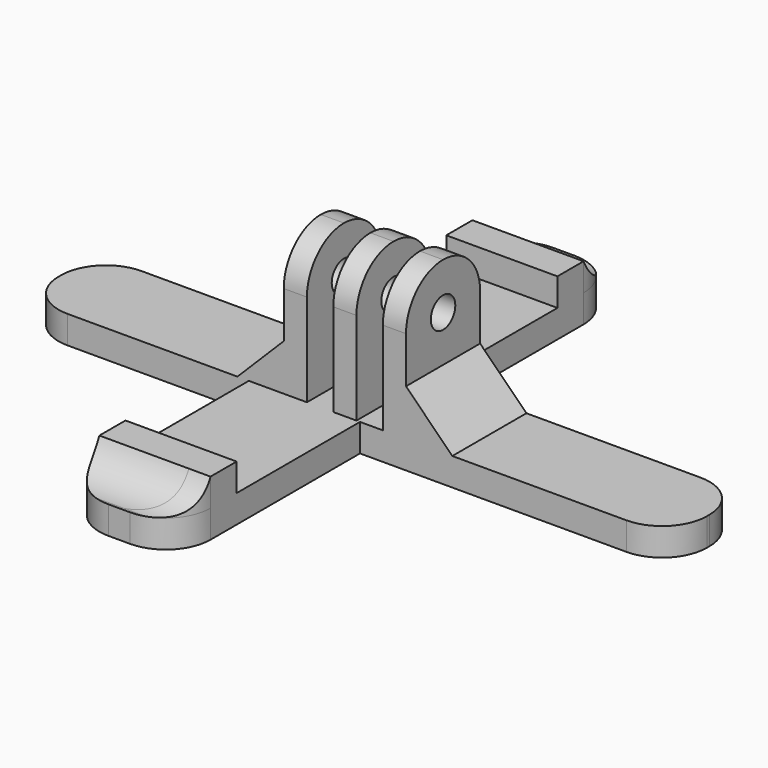
from build123d import *

# Parameters (mm, degrees)
F0_W          = 12
F0_H          = 25
F1_DEPTH      = 3
F2_W          = 2.5
F2_H          = 10
F3_DEPTH      = 15
F5_D          = 3.3
F6_R          = 4.99999
F7_R          = 4.8284271247
F8_T1_DEPTH   = 10
F9_W          = 12
F9_H          = 3.5225884728
F10_DEPTH     = 3
F11_T3_DEPTH  = 34.9128784748
F11_S4_R      = 4.8284271247
F11_T5_DEPTH  = 19
F11_T8_DEPTH  = 34.9128784748
F11_S9_R      = 4.8284271247
F11_T10_DEPTH = 19
F11_T13_DEPTH = 34.9128784748
F11_S14_R     = 4.8284271247
F11_T15_DEPTH = 19
F11_T18_DEPTH = 34.9128784748
F11_S19_R     = 4.8284271247
F11_T20_DEPTH = 19


# Not quite as in the source:
# - a fillet or chamfer that OpenCascade refuses, or shapes differently, is made with other operations: its cross-section is extruded or revolved along the edge and cut away or added
# - a fillet or chamfer is up to 0.001 mm smaller than in the source, because OpenCascade refuses the exact size


with BuildPart() as f1:
    # F0 (on Top) → F1 (new body)
    with BuildSketch(Plane.XY):
        Polygon((35, -5), (35, 5), (1.4061683491, 5), (-10.5938316509, 5), (-35, 5), (-35, -5), (-10.5938316509, -5), (1.4061683491, -5), align=None)
        with Locations((-4.5938316509, 17.5)):
            Rectangle(F0_W, F0_H)
        with Locations((-4.5938316509, -17.5)):
            Rectangle(F0_W, F0_H)
    extrude(amount=F1_DEPTH)

    # F2 (on face) → F3 (join)
    with BuildSketch(Plane.XY.offset(3)):
        with Locations((-5.5737404495, 0)):
            Rectangle(F2_W, F2_H)
        with Locations((-0.2237404495, 0)):
            Rectangle(F2_W, F2_H)
        with Locations((5.1262595505, 0)):
            Rectangle(F2_W, F2_H)
    extrude(amount=F3_DEPTH)

    # F5 (through all)
    with Locations(Plane.YZ.offset(6.3762595505)):
        with Locations((0, 12.9813589156)):
            Hole(F5_D / 2)

    # F6 (radius 5 in the source; OpenCascade refuses exactly that, so slightly less here)
    f6_edges = [f1.edges().sort_by_distance(p)[0] for p in [
        (5.12626, 5, 18),
        (-0.22374, 5, 18),
        (-5.57374, 5, 18),
        (-5.57374, -5, 18),
        (-0.22374, -5, 18),
        (5.12626, -5, 18),
    ]]
    fillet(f6_edges, radius=F6_R)

    # F7
    f7_edges = [f1.edges().sort_by_distance(p)[0] for p in [
        (35, 5, 1.5),
        (35, -5, 1.5),
        (-35, -5, 1.5),
        (-35, 5, 1.5),
        (-10.593832, -30, 1.5),
        (1.406168, -30, 1.5),
        (1.406168, 30, 1.5),
        (-10.593832, 30, 1.5),
    ]]
    fillet(f7_edges, radius=F7_R)

    # F8: chamfer of 5 on 2 edges, made by hand

    # F8_s2 → F8_t1 (join)
    with BuildSketch(Plane.XZ.offset(-5)):
        Polygon((11.3762595505, 3), (6.3762595505, 8), (6.3762595505, 3), align=None)
        Polygon((-11.8237404495, 3), (-6.8237404495, 8), (-6.8237404495, 3), align=None)
    extrude(amount=F8_T1_DEPTH)

    # F9 (on face) → F10 (join)
    with BuildSketch(Plane.XY.offset(3)):
        with Locations((-4.5938316509, 23.4102786388)):
            Rectangle(F9_W, F9_H)
        with Locations((-4.5938316509, -23.4102786388)):
            Rectangle(F9_W, F9_H)
    extrude(amount=F10_DEPTH)

    # F11: fillet of radius 5 on 2 edges, made by hand


with BuildPart() as f11_tool1:
    # F11_s2 → F11_t3 (new body)
    with BuildSketch(Plane.YZ.offset(-22.0502708883)):
        with BuildLine():
            ThreePointArc((-29.7541485702, 3), (-27.0155357827, 3.8166998673), (-25.1715728753, 6))
            Line((-25.1715728753, 6), (-25.1715728753, 3))
            Line((-25.1715728753, 3), (-29.7541485702, 3))
        make_face()
    extrude(amount=F11_T3_DEPTH)

    # F11_s4 → F11_t5 (intersect, symmetric)
    with BuildSketch(Plane.XY.offset(4.5)):
        with Locations((-5.7654045262, -25.1715728753)):
            Circle(F11_S4_R)
    extrude(amount=F11_T5_DEPTH, both=True, mode=Mode.INTERSECT)


with BuildPart() as f11_tool6:
    # F11_s7 → F11_t8 (new body)
    with BuildSketch(Plane.YZ.offset(-22.0502708883)):
        with BuildLine():
            ThreePointArc((-29.7541485702, 3), (-27.0155357827, 3.8166998673), (-25.1715728753, 6))
            Line((-25.1715728753, 6), (-25.1715728753, 3))
            Line((-25.1715728753, 3), (-29.7541485702, 3))
        make_face()
    extrude(amount=F11_T8_DEPTH)

    # F11_s9 → F11_t10 (intersect, symmetric)
    with BuildSketch(Plane.XY.offset(4.5)):
        with Locations((-3.4222587757, -25.1715728753)):
            Circle(F11_S9_R)
    extrude(amount=F11_T10_DEPTH, both=True, mode=Mode.INTERSECT)


with BuildPart() as f11_tool11:
    # F11_s12 → F11_t13 (new body)
    with BuildSketch(Plane.YZ.offset(12.8626075865)):
        with BuildLine():
            ThreePointArc((29.7541485702, 3), (27.0155357827, 3.8166998673), (25.1715728753, 6))
            Line((25.1715728753, 6), (25.1715728753, 3))
            Line((25.1715728753, 3), (29.7541485702, 3))
        make_face()
    extrude(amount=-F11_T13_DEPTH)

    # F11_s14 → F11_t15 (intersect, symmetric)
    with BuildSketch(Plane.XY.offset(4.5)):
        with Locations((-3.4222587757, 25.1715728753)):
            Circle(F11_S14_R)
    extrude(amount=F11_T15_DEPTH, both=True, mode=Mode.INTERSECT)


with BuildPart() as f11_tool16:
    # F11_s17 → F11_t18 (new body)
    with BuildSketch(Plane.YZ.offset(12.8626075865)):
        with BuildLine():
            ThreePointArc((29.7541485702, 3), (27.0155357827, 3.8166998673), (25.1715728753, 6))
            Line((25.1715728753, 6), (25.1715728753, 3))
            Line((25.1715728753, 3), (29.7541485702, 3))
        make_face()
    extrude(amount=-F11_T18_DEPTH)

    # F11_s19 → F11_t20 (intersect, symmetric)
    with BuildSketch(Plane.XY.offset(4.5)):
        with Locations((-5.7654045262, 25.1715728753)):
            Circle(F11_S19_R)
    extrude(amount=F11_T20_DEPTH, both=True, mode=Mode.INTERSECT)


with BuildPart() as f1_1:
    add(f1.part)

    # F11_t21: union F11_tool1, F11_tool6, F11_tool11, F11_tool16
    add([f11_tool1.part, f11_tool6.part, f11_tool11.part, f11_tool16.part])


solid = f1_1.part
